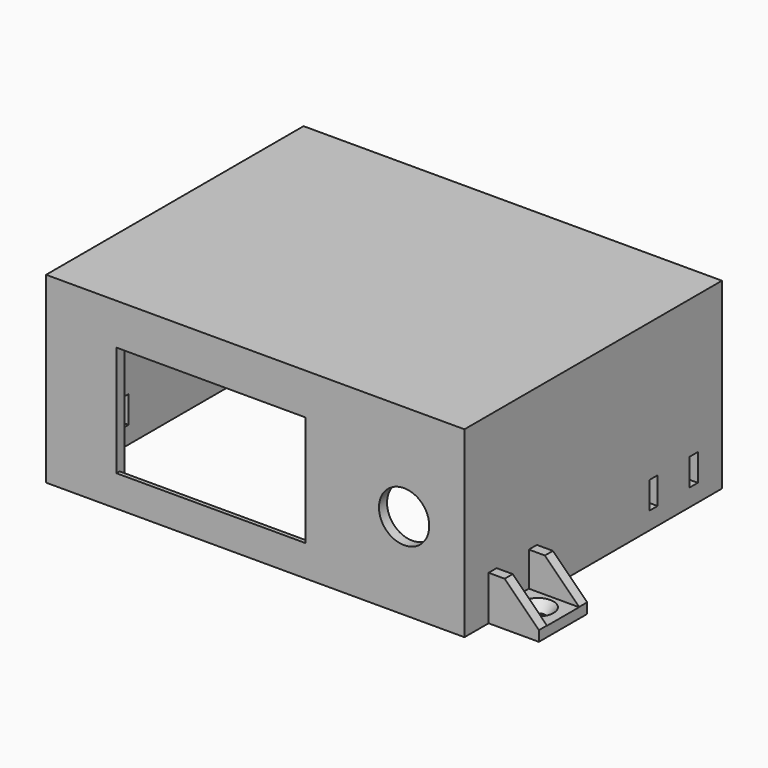
from build123d import *

# Parameters (mm, degrees)
F2_DEPTH        = 80
F1_W            = 99
F1_H            = 43
F1_W_2          = 47
F1_H_2          = 27.5
F1_R            = 6.25
F3_DEPTH        = 2.5
F4_R            = 1.75
F5_DEPTH        = 5
F6_W            = 2.5
F6_H            = 6.7354051862
F6_W_2          = 2.1
F6_H_2          = 6.3354051862
F7_DEPTH        = 104
F8_DEPTH        = 12.5
F9_DEPTH        = 4
F10_SIZE        = 8.5
F12_D           = 3.7973
F12_CSINK_D     = 7.7978
F12_CSINK_ANGLE = 82
F14_DEPTH       = 2
F15_W           = 47
F15_H           = 1.5
F16_DEPTH       = 2


with BuildPart() as f2:
    # F1 (on Front) → F2 (new body)
    with BuildSketch(Plane.XZ):
        Polygon((-15, -7.75), (-15, 35.25), (84, 35.25), (84, -7.75), (86.5, -7.75), (86.5, 37.75), (-17.5, 37.75), (-17.5, -7.75), align=None)
    extrude(amount=-F2_DEPTH)

    # F1 (on Front) → F3 (join)
    with BuildSketch(Plane.XZ):
        with Locations((34.5, 13.75)):
            Rectangle(F1_W, F1_H)
        with Locations((23.5, 13.75)):
            Rectangle(F1_W_2, F1_H_2, mode=Mode.SUBTRACT)
        with Locations((71.5, 13.75)):
            Circle(F1_R, mode=Mode.SUBTRACT)
    extrude(amount=-F3_DEPTH)

    # F4 (on face) → F5 (join)
    with BuildSketch(Plane(origin=(0, 0, 35.25), x_dir=(1, 0, 0), z_dir=(0, 0, -1))):
        with Locations((-9.5, -75)):
            Circle(F4_R)
        with Locations((74.5, -75)):
            Circle(F4_R)
    extrude(amount=F5_DEPTH)

    # F6 (on face) → F7 (cut, through all)
    with BuildSketch(Plane.YZ.offset(86.5)):
        with Locations((8.75, -0.0630606664)):
            Rectangle(F6_W, F6_H)
        with Locations((8.75, -0.0630606664)):
            Rectangle(F6_W_2, F6_H_2, mode=Mode.SUBTRACT)
        with Locations((21.25, -0.0630606664)):
            Rectangle(F6_W, F6_H)
        with Locations((21.25, -0.0630606664)):
            Rectangle(F6_W_2, F6_H_2, mode=Mode.SUBTRACT)
        with Locations((58.75, -0.0630606664)):
            Rectangle(F6_W, F6_H)
        with Locations((71.25, -0.0630606664)):
            Rectangle(F6_W, F6_H)
        with Locations((8.75, -0.0630606664)):
            Rectangle(F6_W_2, F6_H_2)
        with Locations((21.25, -0.0630606664)):
            Rectangle(F6_W_2, F6_H_2)
    extrude(amount=-F7_DEPTH, mode=Mode.SUBTRACT)

    # F13 (on face) → F14 (cut)
    with BuildSketch(Plane.XY):
        Polygon((47, 2.5), (0, 2.5), (0, 1), (47, 1), (47, 1.25), align=None)
    extrude(amount=-F14_DEPTH, mode=Mode.SUBTRACT)

    # F15 (on face) → F16 (cut)
    with BuildSketch(Plane(origin=(0, 0, 27.5), x_dir=(1, 0, 0), z_dir=(0, 0, -1))):
        with Locations((23.5, -1.75)):
            Rectangle(F15_W, F15_H)
    extrude(amount=-F16_DEPTH, mode=Mode.SUBTRACT)


with BuildPart() as f8:
    # F6 (on face) → F8 (new body)
    with BuildSketch(Plane.YZ.offset(86.5)):
        with Locations((8.75, -0.0630606664)):
            Rectangle(F6_W, F6_H)
        with Locations((8.75, -0.0630606664)):
            Rectangle(F6_W_2, F6_H_2, mode=Mode.SUBTRACT)
        Polygon((7.5, -3.4307632595), (7.5, -7.75), (15, -7.75), (22.5, -7.75), (22.5, -3.4307632595), (20, -3.4307632595), (20, -5.25), (15, -5.25), (10, -5.25), (10, -3.4307632595), align=None)
        with Locations((21.25, -0.0630606664)):
            Rectangle(F6_W, F6_H)
        with Locations((21.25, -0.0630606664)):
            Rectangle(F6_W_2, F6_H_2, mode=Mode.SUBTRACT)
        with Locations((8.75, -0.0630606664)):
            Rectangle(F6_W_2, F6_H_2)
        with Locations((21.25, -0.0630606664)):
            Rectangle(F6_W_2, F6_H_2)
    extrude(amount=F8_DEPTH)

    # F6 (on face) → F9 (join)
    with BuildSketch(Plane.YZ.offset(86.5)):
        with Locations((8.75, -0.0630606664)):
            Rectangle(F6_W_2, F6_H_2)
        with Locations((21.25, -0.0630606664)):
            Rectangle(F6_W_2, F6_H_2)
    extrude(amount=-F9_DEPTH)

    # F10
    f10_edges = [f8.edges().sort_by_distance(p)[0] for p in [
        (99, 8.75, 3.304642),
        (99, 21.25, 3.304642),
    ]]
    chamfer(f10_edges, length=F10_SIZE)

    # F12 (through all)
    with Locations(Plane.XY.offset(-5.25)):
        with Locations((92.75, 15)):
            CounterSinkHole(F12_D / 2, F12_CSINK_D / 2, counter_sink_angle=F12_CSINK_ANGLE)


solid = Compound([f2.part, f8.part])
